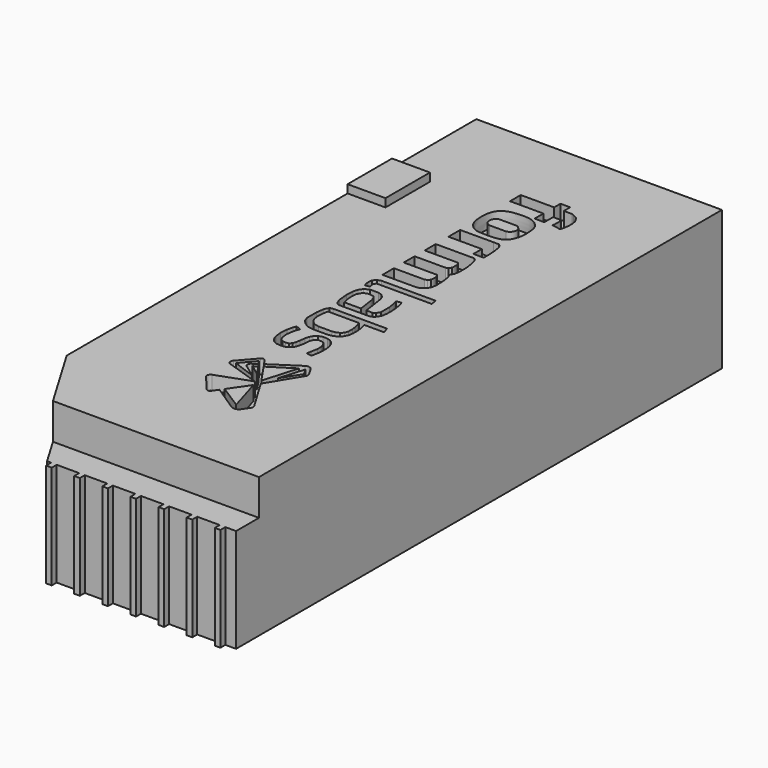
from build123d import *

# Parameters (mm, degrees)
F1_DEPTH  = 13.208
F3_DEPTH  = 4.572
F4_W      = 4.8257596791
F4_H      = 7.0775784552
F5_DEPTH  = 1.0414
F6_W      = 1.3165149344
F6_H      = 3.32568679
F7_DEPTH  = 1.524
F8_W      = 2.8443624378
F8_H      = 5.0757052377
F10_DEPTH = 1.27
F11_W     = 2.1566674113
F11_H     = 3.3890483901
F11_W_2   = 4.0869903751
F11_H_2   = 5.5913808756
F12_DEPTH = 1.27
F13_W     = 2.1566674113
F13_H     = 3.3890483901
F14_DEPTH = 1.27
F15_W     = 0.7165409625
F15_H     = 13.208
F16_DEPTH = 0.7874
F19_DEPTH = 1.8034


# Not quite as in the source:
# - the program builds the solid bodies; features that only make, move or delete a surface that nothing else refers to are left out


with BuildPart() as f1:
    # F0 (on Top) → F1 (new body)
    with BuildSketch(Plane.XY):
        Polygon((-16.51234366, 29.0305074304), (-16.51234366, -36.1909158528), (-9.3076536432, -48.3251363039), (14.7711858153, -48.3251363039), (14.7711858153, 29.0305074304), align=None)
    extrude(amount=F1_DEPTH)

    # F2 (on face) → F3 (join)
    with BuildSketch(Plane.XY.offset(13.208)):
        Polygon((-11.4724747006, -44.679120183), (14.7711858153, -44.679120183), (14.7711858153, 29.0305074304), (-16.51234366, 29.0305074304), (-16.51234366, -36.1909158528), align=None)
    extrude(amount=F3_DEPTH)

    # F4 (on face) → F5 (join)
    with BuildSketch(Plane.XY.offset(17.78)):
        with Locations((-14.0994638205, 12.0719894767)):
            Rectangle(F4_W, F4_H)
    extrude(amount=F5_DEPTH)

    # F6 (on face) → F7 (cut)
    with BuildSketch(Plane(origin=(-16.51234366, 0, 0), x_dir=(0, -1, 0), z_dir=(-1, 0, 0))):
        with Locations((-26.9439499825, 14.4614572637)):
            Rectangle(F6_W, F6_H)
        with Locations((-24.8611499825, 14.4614572637)):
            Rectangle(F6_W, F6_H)
        with Locations((-22.7783499825, 14.4614572637)):
            Rectangle(F6_W, F6_H)
        with Locations((-24.8433425328, 9.359043395)):
            Rectangle(F6_W, F6_H)
        with Locations((-22.7605425328, 9.359043395)):
            Rectangle(F6_W, F6_H)
        with Locations((-26.9261425328, 9.359043395)):
            Rectangle(F6_W, F6_H)
        with Locations((-24.825535083, 4.2566295264)):
            Rectangle(F6_W, F6_H)
        with Locations((-22.742735083, 4.2566295264)):
            Rectangle(F6_W, F6_H)
        with Locations((-26.908335083, 4.2566295264)):
            Rectangle(F6_W, F6_H)
        with Locations((-20.6701499825, 14.4614572637)):
            Rectangle(F6_W, F6_H)
        with Locations((-16.468935083, 4.2566295264)):
            Rectangle(F6_W, F6_H)
        with Locations((-16.5045499825, 14.4614572637)):
            Rectangle(F6_W, F6_H)
        with Locations((-20.6523425328, 9.359043395)):
            Rectangle(F6_W, F6_H)
        with Locations((-18.5873499825, 14.4614572637)):
            Rectangle(F6_W, F6_H)
        with Locations((-18.5695425328, 9.359043395)):
            Rectangle(F6_W, F6_H)
        with Locations((-16.4867425328, 9.359043395)):
            Rectangle(F6_W, F6_H)
        with Locations((-18.551735083, 4.2566295264)):
            Rectangle(F6_W, F6_H)
        with Locations((-20.634535083, 4.2566295264)):
            Rectangle(F6_W, F6_H)
        with Locations((-14.3963499825, 14.4614572637)):
            Rectangle(F6_W, F6_H)
        with Locations((-10.2307499825, 14.4614572637)):
            Rectangle(F6_W, F6_H)
        with Locations((-14.3785425328, 9.359043395)):
            Rectangle(F6_W, F6_H)
        with Locations((-12.3135499825, 14.4614572637)):
            Rectangle(F6_W, F6_H)
        with Locations((-12.2957425328, 9.359043395)):
            Rectangle(F6_W, F6_H)
        with Locations((-10.2129425328, 9.359043395)):
            Rectangle(F6_W, F6_H)
        with Locations((-5.7171425328, 9.359043395)):
            Rectangle(F6_W, F6_H)
        with Locations((-7.7999425328, 9.359043395)):
            Rectangle(F6_W, F6_H)
        with Locations((-7.8177499825, 14.4614572637)):
            Rectangle(F6_W, F6_H)
        with Locations((-3.6343425328, 9.359043395)):
            Rectangle(F6_W, F6_H)
        with Locations((-5.7349499825, 14.4614572637)):
            Rectangle(F6_W, F6_H)
        with Locations((-3.6521499825, 14.4614572637)):
            Rectangle(F6_W, F6_H)
        with Locations((0.8614574672, 9.359043395)):
            Rectangle(F6_W, F6_H)
        with Locations((-1.2213425328, 9.359043395)):
            Rectangle(F6_W, F6_H)
        with Locations((-1.2391499825, 14.4614572637)):
            Rectangle(F6_W, F6_H)
        with Locations((2.9442574672, 9.359043395)):
            Rectangle(F6_W, F6_H)
        with Locations((0.8436500175, 14.4614572637)):
            Rectangle(F6_W, F6_H)
        with Locations((2.9264500175, 14.4614572637)):
            Rectangle(F6_W, F6_H)
        with Locations((-7.8253425328, 4.406043395)):
            Rectangle(F6_W, F6_H)
        with Locations((0.8360574672, 4.406043395)):
            Rectangle(F6_W, F6_H)
        with Locations((-5.7425425328, 4.406043395)):
            Rectangle(F6_W, F6_H)
        with Locations((2.9188574672, 4.406043395)):
            Rectangle(F6_W, F6_H)
        with Locations((-1.2467425328, 4.406043395)):
            Rectangle(F6_W, F6_H)
        with Locations((-3.6597425328, 4.406043395)):
            Rectangle(F6_W, F6_H)
    extrude(amount=-F7_DEPTH, mode=Mode.SUBTRACT)

    # F8 (on face) → F10 (cut)
    with BuildSketch(Plane(origin=(-16.51234366, 0, 0), x_dir=(0, -1, 0), z_dir=(-1, 0, 0))):
        with Locations((-12.2981038467, 2.5378526188)):
            Rectangle(F8_W, F8_H)
        with BuildLine():
            Line((4.9314470962, 5.1185148768), (4.9314470962, 0))
            Line((4.9314470962, 0), (9.1522773728, 0))
            Line((9.1522773728, 0), (9.1522773728, 5.1185148768))
            ThreePointArc((9.1522773728, 5.1185148768), (7.0418622345, 7.2289300151), (4.9314470962, 5.1185148768))
        make_face()
        with BuildLine():
            ThreePointArc((5.8156104399, 10.9458314255), (5.3735287681, 11.127380532), (4.9314470962, 10.9458314255))
            Line((4.9314470962, 10.9458314255), (4.9314470962, 8.1124510616))
            Line((4.9314470962, 8.1124510616), (5.8156104399, 8.1124510616))
            Line((5.8156104399, 8.1124510616), (5.8156104399, 10.9458314255))
        make_face()
        with BuildLine():
            Line((9.1522773728, 8.1124510616), (9.1522773728, 10.9458314255))
            ThreePointArc((9.1522773728, 10.9458314255), (8.7101957009, 11.127380532), (8.268114029, 10.9458314255))
            Line((8.268114029, 10.9458314255), (8.268114029, 8.1124510616))
            Line((8.268114029, 8.1124510616), (9.1522773728, 8.1124510616))
        make_face()
        Polygon((6.1025461182, 16.1243006587), (4.6088052914, 16.1246620119), (4.6088052914, 12.8271598369), (6.1025461182, 12.8271598369), align=None)
        Polygon((9.4749191776, 16.1246620119), (7.9811783507, 16.1243006587), (7.9811783507, 12.8271598369), (9.4749191776, 12.8271598369), align=None)
    extrude(amount=-F10_DEPTH, mode=Mode.SUBTRACT)

    # F11 (on face) → F12 (cut)
    with BuildSketch(Plane(origin=(-16.51234366, 0, 0), x_dir=(0, -1, 0), z_dir=(-1, 0, 0))):
        with BuildLine():
            Line((10.4812979698, 10.7828982527), (10.4812979698, 8.2481643185))
            Line((10.4812979698, 8.2481643185), (11.3142484492, 8.2481643185))
            Line((11.3142484492, 8.2481643185), (11.3154808059, 8.2481643185))
            Line((11.3154808059, 8.2481643185), (11.3154808059, 10.7828982527))
            ThreePointArc((11.3154808059, 10.7828982527), (10.8983893879, 11.060843864), (10.4812979698, 10.7828982527))
        make_face()
        with BuildLine():
            Line((12.5854808059, 8.2481643185), (12.5854808059, 10.7828982527))
            ThreePointArc((12.5854808059, 10.7828982527), (12.1683893879, 11.060843864), (11.7512979698, 10.7828982527))
            Line((11.7512979698, 10.7828982527), (11.7512979698, 8.2481643185))
            Line((11.7512979698, 8.2481643185), (12.5854808059, 8.2481643185))
        make_face()
        with BuildLine():
            Line((13.8554808059, 8.2481643185), (13.8554808059, 10.7828982527))
            ThreePointArc((13.8554808059, 10.7828982527), (13.4383893879, 11.060843864), (13.0212979698, 10.7828982527))
            Line((13.0212979698, 10.7828982527), (13.0212979698, 8.2481643185))
            Line((13.0212979698, 8.2481643185), (13.8554808059, 8.2481643185))
        make_face()
        with Locations((12.1677732095, 14.5237841643)):
            Rectangle(F11_W, F11_H)
        with BuildLine():
            ThreePointArc((13.5190375149, 6.1544026248), (12.2032584485, 7.1942196249), (10.9009836305, 6.1375388576))
            Line((10.9009836305, 6.1375388576), (10.9009836305, 2.5078760227))
            Line((10.9009836305, 2.5078760227), (13.5190375149, 2.5078760227))
            Line((13.5190375149, 2.5078760227), (13.5190375149, 6.1544026248))
        make_face()
        with BuildLine():
            Line((17.2122979698, 10.7828982527), (17.2122979698, 8.2481643185))
            Line((17.2122979698, 8.2481643185), (18.0464808059, 8.2481643185))
            Line((18.0464808059, 8.2481643185), (18.0464808059, 10.7828982527))
            ThreePointArc((18.0464808059, 10.7828982527), (17.6293893879, 11.060843864), (17.2122979698, 10.7828982527))
        make_face()
        with BuildLine():
            Line((15.9422979698, 8.2481643185), (16.7764808059, 8.2481643185))
            Line((16.7764808059, 8.2481643185), (16.7764808059, 10.7828982527))
            ThreePointArc((16.7764808059, 10.7828982527), (16.3593893879, 11.060843864), (15.9422979698, 10.7828982527))
            Line((15.9422979698, 10.7828982527), (15.9422979698, 8.2481643185))
        make_face()
        with BuildLine():
            Line((15.5064808059, 8.2481643185), (15.5064808059, 10.7828982527))
            ThreePointArc((15.5064808059, 10.7828982527), (15.0893893879, 11.060843864), (14.6722979698, 10.7828982527))
            Line((14.6722979698, 10.7828982527), (14.6722979698, 8.2481643185))
            Line((14.6722979698, 8.2481643185), (15.5052484492, 8.2481643185))
            Line((15.5052484492, 8.2481643185), (15.5064808059, 8.2481643185))
        make_face()
        with BuildLine():
            Line((15.0919836305, 6.1375388576), (15.0919836305, 2.5078760227))
            Line((15.0919836305, 2.5078760227), (17.7100375149, 2.5078760227))
            Line((17.7100375149, 2.5078760227), (17.7100375149, 6.1544026248))
            ThreePointArc((17.7100375149, 6.1544026248), (16.3942584485, 7.1942196249), (15.0919836305, 6.1375388576))
        make_face()
        with Locations((16.3587732095, 14.5237841643)):
            Rectangle(F11_W, F11_H)
        with BuildLine():
            Line((21.4032979698, 10.7828982527), (21.4032979698, 8.2481643185))
            Line((21.4032979698, 8.2481643185), (22.2374808059, 8.2481643185))
            Line((22.2374808059, 8.2481643185), (22.2374808059, 10.7828982527))
            ThreePointArc((22.2374808059, 10.7828982527), (21.8203893879, 11.060843864), (21.4032979698, 10.7828982527))
        make_face()
        with BuildLine():
            Line((20.1332979698, 8.2481643185), (20.9674808059, 8.2481643185))
            Line((20.9674808059, 8.2481643185), (20.9674808059, 10.7828982527))
            ThreePointArc((20.9674808059, 10.7828982527), (20.5503893879, 11.060843864), (20.1332979698, 10.7828982527))
            Line((20.1332979698, 10.7828982527), (20.1332979698, 8.2481643185))
        make_face()
        with BuildLine():
            Line((19.6974808059, 8.2481643185), (19.6974808059, 10.7828982527))
            ThreePointArc((19.6974808059, 10.7828982527), (19.2803893879, 11.060843864), (18.8632979698, 10.7828982527))
            Line((18.8632979698, 10.7828982527), (18.8632979698, 8.2481643185))
            Line((18.8632979698, 8.2481643185), (19.6962484492, 8.2481643185))
            Line((19.6962484492, 8.2481643185), (19.6974808059, 8.2481643185))
        make_face()
        with BuildLine():
            Line((19.2829836305, 6.1375388576), (19.2829836305, 2.5078760227))
            Line((19.2829836305, 2.5078760227), (21.9010375149, 2.5078760227))
            Line((21.9010375149, 2.5078760227), (21.9010375149, 6.1544026248))
            ThreePointArc((21.9010375149, 6.1544026248), (20.5852584485, 7.1942196249), (19.2829836305, 6.1375388576))
        make_face()
        with Locations((20.5497732095, 14.5237841643)):
            Rectangle(F11_W, F11_H)
        with BuildLine():
            Line((25.5942979698, 10.7828982527), (25.5942979698, 8.2481643185))
            Line((25.5942979698, 8.2481643185), (26.4284808059, 8.2481643185))
            Line((26.4284808059, 8.2481643185), (26.4284808059, 10.7828982527))
            ThreePointArc((26.4284808059, 10.7828982527), (26.0113893879, 11.060843864), (25.5942979698, 10.7828982527))
        make_face()
        with BuildLine():
            Line((24.3242979698, 8.2481643185), (25.1584808059, 8.2481643185))
            Line((25.1584808059, 8.2481643185), (25.1584808059, 10.7828982527))
            ThreePointArc((25.1584808059, 10.7828982527), (24.7413893879, 11.060843864), (24.3242979698, 10.7828982527))
            Line((24.3242979698, 10.7828982527), (24.3242979698, 8.2481643185))
        make_face()
        with BuildLine():
            Line((23.8884808059, 8.2481643185), (23.8884808059, 10.7828982527))
            ThreePointArc((23.8884808059, 10.7828982527), (23.4713893879, 11.060843864), (23.0542979698, 10.7828982527))
            Line((23.0542979698, 10.7828982527), (23.0542979698, 8.2481643185))
            Line((23.0542979698, 8.2481643185), (23.8872484492, 8.2481643185))
            Line((23.8872484492, 8.2481643185), (23.8884808059, 8.2481643185))
        make_face()
        with Locations((24.7407732095, 14.5237841643)):
            Rectangle(F11_W, F11_H)
        with BuildLine():
            Line((29.7852979698, 10.7828982527), (29.7852979698, 8.2481643185))
            Line((29.7852979698, 8.2481643185), (30.6194808059, 8.2481643185))
            Line((30.6194808059, 8.2481643185), (30.6194808059, 10.7828982527))
            ThreePointArc((30.6194808059, 10.7828982527), (30.2023893879, 11.060843864), (29.7852979698, 10.7828982527))
        make_face()
        with BuildLine():
            Line((28.5152979698, 8.2481643185), (29.3494808059, 8.2481643185))
            Line((29.3494808059, 8.2481643185), (29.3494808059, 10.7828982527))
            ThreePointArc((29.3494808059, 10.7828982527), (28.9323893879, 11.060843864), (28.5152979698, 10.7828982527))
            Line((28.5152979698, 10.7828982527), (28.5152979698, 8.2481643185))
        make_face()
        with BuildLine():
            Line((28.0794808059, 8.2481643185), (28.0794808059, 10.7828982527))
            ThreePointArc((28.0794808059, 10.7828982527), (27.6623893879, 11.060843864), (27.2452979698, 10.7828982527))
            Line((27.2452979698, 10.7828982527), (27.2452979698, 8.2481643185))
            Line((27.2452979698, 8.2481643185), (28.0782484492, 8.2481643185))
            Line((28.0782484492, 8.2481643185), (28.0794808059, 8.2481643185))
        make_face()
        with BuildLine():
            Line((27.6649836305, 6.1375388576), (27.6649836305, 2.5078760227))
            Line((27.6649836305, 2.5078760227), (30.2830375149, 2.5078760227))
            Line((30.2830375149, 2.5078760227), (30.2830375149, 6.1544026248))
            ThreePointArc((30.2830375149, 6.1544026248), (28.9672584485, 7.1942196249), (27.6649836305, 6.1375388576))
        make_face()
        with Locations((28.9317732095, 14.5237841643)):
            Rectangle(F11_W, F11_H)
        with BuildLine():
            Line((33.9762979698, 10.7828982527), (33.9762979698, 8.2481643185))
            Line((33.9762979698, 8.2481643185), (34.8104808059, 8.2481643185))
            Line((34.8104808059, 8.2481643185), (34.8104808059, 10.7828982527))
            ThreePointArc((34.8104808059, 10.7828982527), (34.3933893879, 11.060843864), (33.9762979698, 10.7828982527))
        make_face()
        with BuildLine():
            Line((32.7062979698, 8.2481643185), (33.5404808059, 8.2481643185))
            Line((33.5404808059, 8.2481643185), (33.5404808059, 10.7828982527))
            ThreePointArc((33.5404808059, 10.7828982527), (33.1233893879, 11.060843864), (32.7062979698, 10.7828982527))
            Line((32.7062979698, 10.7828982527), (32.7062979698, 8.2481643185))
        make_face()
        with BuildLine():
            Line((32.2704808059, 8.2481643185), (32.2704808059, 10.7828982527))
            ThreePointArc((32.2704808059, 10.7828982527), (31.8533893879, 11.060843864), (31.4362979698, 10.7828982527))
            Line((31.4362979698, 10.7828982527), (31.4362979698, 8.2481643185))
            Line((31.4362979698, 8.2481643185), (32.2692484492, 8.2481643185))
            Line((32.2692484492, 8.2481643185), (32.2704808059, 8.2481643185))
        make_face()
        with BuildLine():
            Line((31.8559836305, 6.1375388576), (31.8559836305, 2.5078760227))
            Line((31.8559836305, 2.5078760227), (34.4740375149, 2.5078760227))
            Line((34.4740375149, 2.5078760227), (34.4740375149, 6.1544026248))
            ThreePointArc((34.4740375149, 6.1544026248), (33.1582584485, 7.1942196249), (31.8559836305, 6.1375388576))
        make_face()
        with Locations((33.1227732095, 14.5237841643)):
            Rectangle(F11_W, F11_H)
        with Locations((24.7150918003, 2.7956904378)):
            Rectangle(F11_W_2, F11_H_2)
    extrude(amount=-F12_DEPTH, mode=Mode.SUBTRACT)

    # F13 (on face) → F14 (cut)
    with BuildSketch(Plane(origin=(-28.095823784, -16.6818875548, 0), x_dir=(0.5105385773, -0.8598548489, 0), z_dir=(-0.8598548489, -0.5105385773, 0))):
        with BuildLine():
            Line((26.3206895133, 10.9860163945), (26.3206895133, 8.4512824603))
            Line((26.3206895133, 8.4512824603), (27.1548723494, 8.4512824603))
            Line((27.1548723494, 8.4512824603), (27.1548723494, 10.9860163945))
            ThreePointArc((27.1548723494, 10.9860163945), (26.7377809314, 11.2639620058), (26.3206895133, 10.9860163945))
        make_face()
        with BuildLine():
            Line((25.0506895133, 8.4512824603), (25.8848723494, 8.4512824603))
            Line((25.8848723494, 8.4512824603), (25.8848723494, 10.9860163945))
            ThreePointArc((25.8848723494, 10.9860163945), (25.4677809314, 11.2639620058), (25.0506895133, 10.9860163945))
            Line((25.0506895133, 10.9860163945), (25.0506895133, 8.4512824603))
        make_face()
        with BuildLine():
            Line((24.6148723494, 8.4512824603), (24.6148723494, 10.9860163945))
            ThreePointArc((24.6148723494, 10.9860163945), (24.1977809314, 11.2639620058), (23.7806895133, 10.9860163945))
            Line((23.7806895133, 10.9860163945), (23.7806895133, 8.4512824603))
            Line((23.7806895133, 8.4512824603), (24.6136399927, 8.4512824603))
            Line((24.6136399927, 8.4512824603), (24.6148723494, 8.4512824603))
        make_face()
        with BuildLine():
            Line((24.200375174, 6.3406569994), (24.200375174, 2.7109941645))
            Line((24.200375174, 2.7109941645), (26.8184290584, 2.7109941645))
            Line((26.8184290584, 2.7109941645), (26.8184290584, 6.3575207666))
            ThreePointArc((26.8184290584, 6.3575207666), (25.5026499919, 7.3973377667), (24.200375174, 6.3406569994))
        make_face()
        with Locations((25.467164753, 14.7269023061)):
            Rectangle(F13_W, F13_H)
        with BuildLine():
            Line((30.5116895133, 10.9860163945), (30.5116895133, 8.4512824603))
            Line((30.5116895133, 8.4512824603), (31.3458723494, 8.4512824603))
            Line((31.3458723494, 8.4512824603), (31.3458723494, 10.9860163945))
            ThreePointArc((31.3458723494, 10.9860163945), (30.9287809314, 11.2639620058), (30.5116895133, 10.9860163945))
        make_face()
        with BuildLine():
            Line((29.2416895133, 8.4512824603), (30.0758723494, 8.4512824603))
            Line((30.0758723494, 8.4512824603), (30.0758723494, 10.9860163945))
            ThreePointArc((30.0758723494, 10.9860163945), (29.6587809314, 11.2639620058), (29.2416895133, 10.9860163945))
            Line((29.2416895133, 10.9860163945), (29.2416895133, 8.4512824603))
        make_face()
        with BuildLine():
            Line((28.8058723494, 8.4512824603), (28.8058723494, 10.9860163945))
            ThreePointArc((28.8058723494, 10.9860163945), (28.3887809314, 11.2639620058), (27.9716895133, 10.9860163945))
            Line((27.9716895133, 10.9860163945), (27.9716895133, 8.4512824603))
            Line((27.9716895133, 8.4512824603), (28.8046399927, 8.4512824603))
            Line((28.8046399927, 8.4512824603), (28.8058723494, 8.4512824603))
        make_face()
        with BuildLine():
            Line((28.391375174, 6.3406569994), (28.391375174, 2.7109941645))
            Line((28.391375174, 2.7109941645), (31.0094290584, 2.7109941645))
            Line((31.0094290584, 2.7109941645), (31.0094290584, 6.3575207666))
            ThreePointArc((31.0094290584, 6.3575207666), (29.6936499919, 7.3973377667), (28.391375174, 6.3406569994))
        make_face()
        with Locations((29.658164753, 14.7269023061)):
            Rectangle(F13_W, F13_H)
        with BuildLine():
            Line((33.9152895133, 8.4512824603), (34.7494723494, 8.4512824603))
            Line((34.7494723494, 8.4512824603), (34.7494723494, 10.9860163945))
            ThreePointArc((34.7494723494, 10.9860163945), (34.3323809314, 11.2639620058), (33.9152895133, 10.9860163945))
            Line((33.9152895133, 10.9860163945), (33.9152895133, 8.4512824603))
        make_face()
        with BuildLine():
            Line((33.4794723494, 8.4512824603), (33.4794723494, 10.9860163945))
            ThreePointArc((33.4794723494, 10.9860163945), (33.0623809314, 11.2639620058), (32.6452895133, 10.9860163945))
            Line((32.6452895133, 10.9860163945), (32.6452895133, 8.4512824603))
            Line((32.6452895133, 8.4512824603), (33.4782399927, 8.4512824603))
            Line((33.4782399927, 8.4512824603), (33.4794723494, 8.4512824603))
        make_face()
        with BuildLine():
            Line((36.0194723494, 8.4512824603), (36.0194723494, 10.9860163945))
            ThreePointArc((36.0194723494, 10.9860163945), (35.6023809314, 11.2639620058), (35.1852895133, 10.9860163945))
            Line((35.1852895133, 10.9860163945), (35.1852895133, 8.4512824603))
            Line((35.1852895133, 8.4512824603), (36.0194723494, 8.4512824603))
        make_face()
        with BuildLine():
            Line((32.2276167572, 5.3568333387), (32.2276167572, 0))
            Line((32.2276167572, 0), (35.6619991362, 0))
            Line((35.6619991362, 0), (35.6619991362, 5.3568333387))
            ThreePointArc((35.6619991362, 5.3568333387), (33.9448079467, 7.0740245283), (32.2276167572, 5.3568333387))
        make_face()
    extrude(amount=-F14_DEPTH, mode=Mode.SUBTRACT)

    # F15 (on face) → F16 (join)
    with BuildSketch(Plane.XZ.offset(48.3251363039)):
        with Locations((-8.4411241114, 6.604)):
            Rectangle(F15_W, F15_H)
        with Locations((-4.8597241114, 6.604)):
            Rectangle(F15_W, F15_H)
        with Locations((-1.2783241114, 6.604)):
            Rectangle(F15_W, F15_H)
        with Locations((2.3030758886, 6.604)):
            Rectangle(F15_W, F15_H)
        with Locations((5.8844758886, 6.604)):
            Rectangle(F15_W, F15_H)
        with Locations((9.4658758886, 6.604)):
            Rectangle(F15_W, F15_H)
        with Locations((13.0472758886, 6.604)):
            Rectangle(F15_W, F15_H)
    extrude(amount=F16_DEPTH)

    # F18 (on face) → F19 (cut)
    with BuildSketch(Plane.XY.offset(17.78)):
        Polygon((3.6496364046, 15.9182846546), (4.7820697577, 15.7247623586), (4.8945541494, 15.9871354699), (5.0173653092, 16.7057888571), (5.0289309584, 17.3270665109), (4.9430923536, 17.9236643016), (4.5267804526, 18.6366252601), (3.88384494, 18.9692601562), (3.6496364046, 19.0285295248), (2.6398904156, 19.0285295248), (2.6398904156, 20.0345292687), (1.3991386249, 20.0345292687), (1.3991386249, 19.0285295248), (-2.8541032225, 19.0285295248), (-2.8541032225, 17.3237994313), (1.3991386249, 17.3237994313), (1.3991386249, 15.9182846546), (2.6398904156, 15.9182846546), (2.6398904156, 17.3237994313), (3.6496364046, 17.3237994313), (3.7266600411, 17.0736424625), (3.7266600411, 16.2072048258), align=None)
        Polygon((2.0760053303, 9.3912277371), (1.3991386249, 9.3929774708), (-2.8541032225, 9.3929774708), (-2.8541032225, 7.521827706), (1.3991386249, 7.521827706), (1.3991386249, 6.1797631542), (2.7034180223, 6.1797631542), (2.7034180223, 7.2495075874), (2.6571587659, 7.877455093), (2.5019007935, 8.8692036868), (2.3607155308, 9.1030858457), (2.240419155, 9.2616891488), align=None)
        Polygon((2.0571425557, 5.4956623353), (1.3991386249, 5.4956623353), (-2.8541032225, 5.4956623353), (-2.8541032225, 3.7391050719), (1.3991386249, 3.7391050719), (1.5840468695, 3.4327930771), (1.6106679116, 3.020973423), (1.5840468695, 2.5446266618), (1.3460278278, 2.2465330549), (1.0969371069, 2.1292280871), (-2.8541032225, 2.1292280871), (-2.8541032225, 0.404976835), (1.3991386249, 0.404976835), (1.5840468695, 0.1076378141), (1.6181210337, -0.3847229474), (1.5721971868, -0.7834957894), (1.3304969762, -1.052481588), (1.0664551519, -1.1678432347), (-2.8541032225, -1.1678432347), (-2.8541032225, -2.982797011), (1.360576342, -2.982797011), (1.7080920402, -2.9285313945), (2.2337561578, -2.6112090861), (2.3830125574, -2.4913835805), (2.633030283, -2.0257164889), (2.7503571473, -1.3893502764), (2.6853630143, 0), (2.5450269794, 0.7611650716), (2.3250598317, 1.1255543171), (2.6108008651, 1.62266546), (2.7207324747, 2.2189207375), (2.7207324747, 3.4572272561), (2.5726098102, 4.4466871768), (2.3296885192, 5.2643250674), align=None)
        Polygon((4.9081709935, -4.8219300807), (4.7478824854, -4.0410414457), (-2.1257621702, -4.0410414457), (-2.5601014495, -4.1887122206), (-2.9155961238, -4.5560565777), (-2.9747029766, -5.119828973), (-2.9155961238, -5.6016268209), (-2.7861734852, -5.8320518583), (-2.2205850109, -5.7398816571), (-2.316944534, -5.4298555478), (-2.316944534, -5.1072603092), (-2.1257621702, -4.8219300807), align=None)
        Polygon((4.9951227872, -12.5460065901), (4.7478824854, -11.7532359436), (-2.131056739, -11.7532359436), (-2.4862398859, -11.8461251259), (-2.7884102892, -12.3852919787), (-2.9306083452, -13.4043768048), (-2.9306083452, -14.89745453), (-2.7410110924, -15.4721708968), (-2.3025674745, -15.9520879388), (-1.7397010233, -16.3194332272), (-0.9990871185, -16.4616312832), (0.8850345621, -16.4616312832), (1.5195941087, -16.3509882987), (2.0762239583, -16.0902887583), (2.4214752484, -15.7027617097), (2.6680834126, -15.1884071529), (2.7455887757, -14.6317770705), (2.7455887757, -13.9694586396), (2.6892211754, -13.4128285572), (2.548302291, -12.8350611776), (2.449659165, -12.5460065901), align=None)
        Polygon((-2.2494250443, -13.0495997146), (-2.131056739, -12.5460065901), (1.8366617151, -12.5460065901), (1.9423508784, -12.8914285451), (2.0762239583, -13.5326096788), (2.1312199533, -14.0258306637), (2.1312199533, -14.63366393), (1.9792616367, -15.0646278635), (1.6822132748, -15.3888557106), (1.1925199069, -15.5790960416), (0.829653698, -15.6425088644), (-0.8825113182, -15.6425088644), (-1.5413074289, -15.4734048992), (-1.9288344774, -15.1528138667), (-2.2282872815, -14.6419834346), (-2.3304533679, -13.8387456536), align=None, mode=Mode.SUBTRACT)
        Polygon((2.5909075048, -7.1460488252), (2.3842398077, -6.4656501636), (1.7365489621, -6.605152972), (1.8995913466, -7.1297238139), (2.0454477053, -7.9902149737), (2.0454477053, -9.375276044), (1.7963359132, -9.7937844694), (1.48743717, -9.9831093103), (0.6902792957, -9.9831093103), (0.2817358763, -7.272772491), (0.12384579, -6.7647785988), (-0.2971558949, -6.3573574584), (-0.764533761, -6.2364675105), (-1.372366678, -6.2364675105), (-1.8705903785, -6.2364675105), (-2.408067463, -6.5551022999), (-2.7476274408, -7.0360731333), (-2.9155961238, -7.6339412481), (-2.9559389222, -8.6241951212), (-2.8413473628, -9.8099671304), (-2.6403113238, -10.4567783541), (-2.3827497859, -10.7060315501), (-2.0292426925, -10.7765207067), (1.6553095775, -10.7765207067), (2.0981925725, -10.638867803), (2.3926305145, -10.3346153787), (2.6467745192, -9.855565615), (2.7364548296, -9.1281589121), (2.7364548296, -8.5751311854), (2.6965970173, -7.8576887026), align=None)
        Polygon((-0.2833141189, -7.9895872623), (0, -9.9831093103), (-2.1257621702, -9.9831093103), (-2.2859165911, -9.1961752623), (-2.3529492319, -8.5593648255), (-2.2775374819, -7.8576887026), (-1.975890249, -7.2941225953), (-1.5317985089, -7.0678866468), (-1.0960858781, -7.0678866468), (-0.6938895094, -7.1516777389), (-0.4341377062, -7.4617043138), align=None, mode=Mode.SUBTRACT)
        Polygon((1.8190216506, -20.9149960428), (2.5060013868, -20.9854561836), (2.6694443077, -20.2245377004), (2.7387277223, -19.4711629301), (2.7387277223, -18.9181342721), (2.659011865, -18.3252487332), (2.4597225711, -17.8320072591), (2.1607882809, -17.468303442), (1.8319606315, -17.2391198575), (1.4483284904, -17.1245280653), (0.8554423111, -17.1245280653), (0.3671832092, -17.2690134495), (0, -17.6127869636), (-0.1708983764, -17.9416146129), (-0.3353121865, -18.4796974063), (-0.4249924386, -19.1522985697), (-0.5096905516, -19.6604859084), (-0.6541753537, -20.0889594853), (-0.8933227509, -20.3181412071), (-1.2620082125, -20.3779283911), (-1.7203737516, -20.3231219202), (-2.0143256988, -20.1188512146), (-2.2086328827, -19.7202712297), (-2.303295536, -18.9978480339), (-2.2335441317, -18.3352101594), (-2.0827232761, -17.7013480796), (-1.9239711564, -17.2364311386), (-2.5872830302, -17.0099344105), (-2.7267856058, -17.4184776843), (-2.8961815406, -18.1259568781), (-2.9808797408, -19.0277416259), (-2.8762526345, -19.9345070869), (-2.6919099037, -20.4327311367), (-2.298313193, -20.9209900349), (-1.8847875763, -21.1501736194), (-1.1872744653, -21.2049782276), (-0.6292639882, -21.1202800274), (-0.086200198, -20.7466129214), (0.1702701411, -20.2033556998), (0.3147120588, -19.4952376187), (0.37107963, -18.7800750136), (0.5472283228, -18.2023067027), (0.9100945317, -17.9416071624), (1.350466162, -17.9416071624), (1.6957175685, -18.0790033191), (1.9669865724, -18.4982363135), (2.086767694, -18.9421307296), (2.086767694, -19.4705780596), (1.9388027722, -20.3196145594), align=None)
        with BuildLine():
            Line((-2.6895201141, -27.4287047059), (1.5871455368, -28.8448039946))
            Line((1.5871455368, -28.8448039946), (-2.6512101482, -30.3771978003))
            ThreePointArc((-2.6512101482, -30.3771978003), (-2.9327331048, -30.6771410081), (-2.8564403938, -31.0813693164))
            Line((-2.8564403938, -31.0813693164), (-1.0924299763, -33.1681410174))
            ThreePointArc((-1.0924299763, -33.1681410174), (-0.8092727719, -33.2912756323), (-0.5394108987, -33.1412266232))
            Line((-0.5394108987, -33.1412266232), (-0.0524890856, -32.4363484979))
            Line((-0.0524890856, -32.4363484979), (3.1679740821, -34.5638773149))
            ThreePointArc((3.1679740821, -34.5638773149), (3.7788465935, -34.6823596156), (4.2949024554, -34.3346677575))
            Line((4.2949024554, -34.3346677575), (4.8129364536, -33.5536819472))
            ThreePointArc((4.8129364536, -33.5536819472), (4.8996472886, -33.2773906094), (4.8254720903, -32.9974732783))
            Line((4.8254720903, -32.9974732783), (2.3328172737, -28.8448039946))
            Line((2.3328172737, -28.8448039946), (4.7956805128, -24.8003706354))
            ThreePointArc((4.7956805128, -24.8003706354), (4.8737914199, -24.5303785154), (4.8045019065, -24.2579890478))
            Line((4.8045019065, -24.2579890478), (4.2880181022, -23.3442070102))
            ThreePointArc((4.2880181022, -23.3442070102), (3.8770986252, -23.0339512227), (3.3698537502, -23.1223599727))
            Line((3.3698537502, -23.1223599727), (-0.0372060967, -25.3652557731))
            Line((-0.0372060967, -25.3652557731), (-0.5179640085, -24.6632397717))
            ThreePointArc((-0.5179640085, -24.6632397717), (-0.7931405555, -24.5077454992), (-1.084551124, -24.6301402758))
            Line((-1.084551124, -24.6301402758), (-2.8889915787, -26.6992622665))
            ThreePointArc((-2.8889915787, -26.6992622665), (-2.9847565593, -27.1174446113), (-2.6895201141, -27.4287047059))
        make_face()
        with BuildLine():
            Line((-0.8522951563, -25.1644581675), (-0.4931872339, -25.6888374896))
            Line((-0.4931872339, -25.6888374896), (-1.0816728143, -26.0918469625))
            ThreePointArc((-1.0816728143, -26.0918469625), (-1.2718780731, -26.4469033124), (-1.0911655927, -26.806883939))
            Line((-1.0911655927, -26.806883939), (0.5578011042, -28.0016567558))
            Line((0.5578011042, -28.0016567558), (-2.366353292, -26.9346237183))
            Line((-2.366353292, -26.9346237183), (-0.8522951563, -25.1644581675))
        make_face(mode=Mode.SUBTRACT)
        Polygon((-0.642499479, -26.416471228), (-0.1642047719, -26.117535308), (0.7425622898, -27.4627394974), align=None, mode=Mode.SUBTRACT)
        Polygon((0.2519718001, -31.9956045989), (1.9543613307, -29.5311901718), (3.2535414796, -33.9092159095), align=None, mode=Mode.SUBTRACT)
        Polygon((0.2693736648, -25.8129320215), (3.2535414796, -23.9104150411), (1.9755434175, -28.3043282904), align=None, mode=Mode.SUBTRACT)
        Polygon((4.3996204622, -24.5689954609), (2.9539421666, -26.861935854), (3.8900780492, -23.6861836165), align=None, mode=Mode.SUBTRACT)
        with BuildLine():
            add(Edge.make_bspline(
                [(2.7912307996, 12.8015707138), (2.7904512528, 12.5023329121), (2.7530806222, 11.7467631778), (2.113413426, 10.3761309911), (0.6472334209, 10.1528456973), (-0.8468334404, 10.1724108772), (-1.7669813008, 10.2885475854), (-2.6114689495, 10.9937050892), (-3.0056931295, 11.9882423284), (-3.0304433307, 13.7037930298), (-2.7094770328, 14.7353291444), (-1.9021511327, 15.4438318816), (-0.6383974612, 15.6832902772), (0.8528925529, 15.7034280293), (1.7164292335, 15.4232202192), (2.6367894788, 14.6412773756), (2.7675425987, 13.5260957539), (2.7918843289, 13.0524352768), (2.7912307996, 12.8015707138)],
                knots=[0, 0, 0, 0, 0.0593890794, 0.1277263015, 0.1965836521, 0.2681821573, 0.3237085605, 0.3820054342, 0.4422383411, 0.5180936465, 0.5781138642, 0.6356594441, 0.7019411555, 0.7727396491, 0.8280755768, 0.8899340238, 0.9502114527, 1, 1, 1, 1], degree=3))
        make_face()
        with BuildLine():
            Line((-1.2244065292, 13.6111658067), (0.9156931192, 13.6111658067))
            ThreePointArc((0.9156931192, 13.6111658067), (1.5845228609, 12.8015707138), (0.9156931192, 11.9919756209))
            ThreePointArc((0.9156931192, 11.9919756209), (0.9108876157, 11.9910669278), (0.9060768061, 11.9901867583))
            Line((0.9060768061, 11.9901867583), (-1.2244065292, 11.9901867583))
            ThreePointArc((-1.2244065292, 11.9901867583), (-1.8631988621, 12.8006762825), (-1.2244065292, 13.6111658067))
        make_face(mode=Mode.SUBTRACT)
    extrude(amount=-F19_DEPTH, mode=Mode.SUBTRACT)


solid = f1.part
